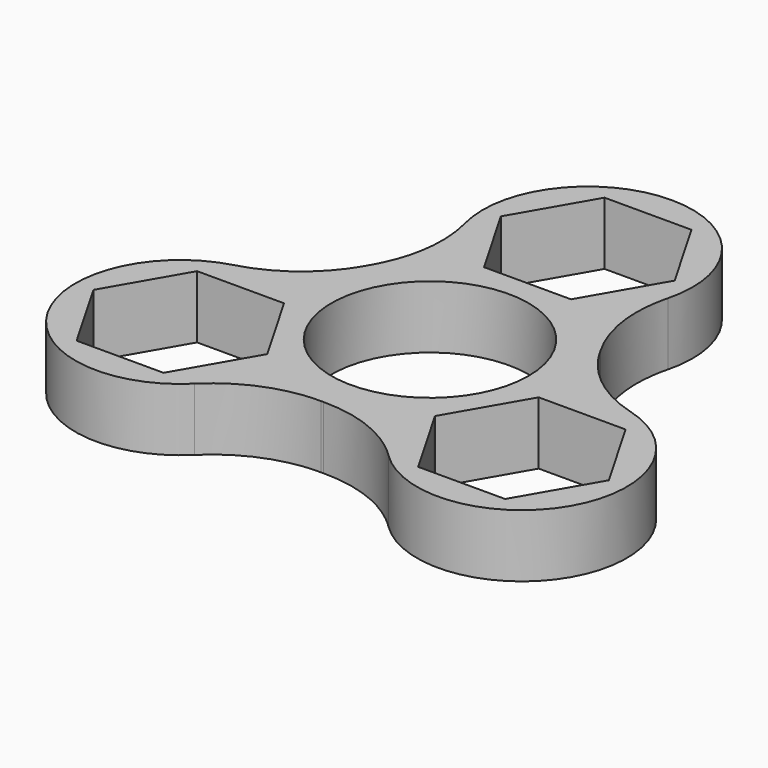
from build123d import *

# Parameters (mm, degrees)
F0_R     = 11
F1_DEPTH = 7
F2_R     = 15


with BuildPart() as f1:
    # F0 (on Top) → F1 (new body)
    with BuildSketch(Plane.XY):
        with BuildLine():
            ThreePointArc((-14.7729482501, -2.6), (-14.9420444362, -1.3173109227), (-14.9999794627, -0.0248217267))
            ThreePointArc((-14.9999794627, -0.0248217267), (-29.1846096908, -16.8497422612), (-7.5214859773, -12.9779524076))
            ThreePointArc((-7.5214859773, -12.9779524076), (-8.6118469419, -12.2815346048), (-9.6381401749, -11.4937484734))
            Line((-9.6381401749, -11.4937484734), (-14.2028166221, -19.4))
            Line((-14.2028166221, -19.4), (-23.9023011445, -19.4))
            Line((-23.9023011445, -19.4), (-28.7520434056, -11))
            Line((-28.7520434056, -11), (-23.9023011445, -2.6))
            Line((-23.9023011445, -2.6), (-14.7729482501, -2.6))
        make_face()
        with BuildLine():
            ThreePointArc((14.9999794627, -0.0248217267), (14.9999948657, -0.0124108676), (15, 0))
            ThreePointArc((15, 0), (12.9841711765, 7.5107455595), (7.4784934854, 13.0027741343))
            ThreePointArc((7.4784934854, 13.0027741343), (6.3301974943, 13.5988455276), (5.1348080752, 14.0937484734))
            Line((5.1348080752, 14.0937484734), (4.8497422612, 13.6))
            Line((4.8497422612, 13.6), (-4.8497422612, 13.6))
            Line((-4.8497422612, 13.6), (-5.1348080752, 14.0937484734))
            ThreePointArc((-5.1348080752, 14.0937484734), (-6.3301974943, 13.5988455276), (-7.4784934854, 13.0027741343))
            ThreePointArc((-7.4784934854, 13.0027741343), (-12.9903810568, 7.5), (-14.9999794627, -0.0248217267))
            ThreePointArc((-14.9999794627, -0.0248217267), (-14.9420444362, -1.3173109227), (-14.7729482501, -2.6))
            Line((-14.7729482501, -2.6), (-14.2028166221, -2.6))
            Line((-14.2028166221, -2.6), (-9.3530743609, -11))
            Line((-9.3530743609, -11), (-9.6381401749, -11.4937484734))
            ThreePointArc((-9.6381401749, -11.4937484734), (-8.6118469419, -12.2815346048), (-7.5214859773, -12.9779524076))
            ThreePointArc((-7.5214859773, -12.9779524076), (0, -15), (7.5214859773, -12.9779524076))
            ThreePointArc((7.5214859773, -12.9779524076), (8.6118469419, -12.2815346048), (9.6381401749, -11.4937484734))
            Line((9.6381401749, -11.4937484734), (9.3530743609, -11))
            Line((9.3530743609, -11), (14.2028166221, -2.6))
            Line((14.2028166221, -2.6), (14.7729482501, -2.6))
            ThreePointArc((14.7729482501, -2.6), (14.9420444362, -1.3173109227), (14.9999794627, -0.0248217267))
        make_face()
        Circle(F0_R, mode=Mode.SUBTRACT)
        with BuildLine():
            ThreePointArc((7.5214859773, -12.9779524076), (29.1846096908, -16.8497422612), (14.9999794627, -0.0248217267))
            ThreePointArc((14.9999794627, -0.0248217267), (14.9420444362, -1.3173109227), (14.7729482501, -2.6))
            Line((14.7729482501, -2.6), (23.9023011445, -2.6))
            Line((23.9023011445, -2.6), (28.7520434056, -11))
            Line((28.7520434056, -11), (23.9023011445, -19.4))
            Line((23.9023011445, -19.4), (14.2028166221, -19.4))
            Line((14.2028166221, -19.4), (9.6381401749, -11.4937484734))
            ThreePointArc((9.6381401749, -11.4937484734), (8.6118469419, -12.2815346048), (7.5214859773, -12.9779524076))
        make_face()
        with BuildLine():
            ThreePointArc((5.1348080752, 14.0937484734), (6.3301974943, 13.5988455276), (7.4784934854, 13.0027741343))
            ThreePointArc((7.4784934854, 13.0027741343), (0, 33.6994845224), (-7.4784934854, 13.0027741343))
            ThreePointArc((-7.4784934854, 13.0027741343), (-6.3301974943, 13.5988455276), (-5.1348080752, 14.0937484734))
            Line((-5.1348080752, 14.0937484734), (-9.6994845224, 22))
            Line((-9.6994845224, 22), (-4.8497422612, 30.4))
            Line((-4.8497422612, 30.4), (4.8497422612, 30.4))
            Line((4.8497422612, 30.4), (9.6994845224, 22))
            Line((9.6994845224, 22), (5.1348080752, 14.0937484734))
        make_face()
    extrude(amount=F1_DEPTH)

    # F2
    f2_edges = [f1.edges().sort_by_distance(p)[0] for p in [
        (7.521486, -12.977952, 3.5),
        (-14.999979, -0.024822, 3.5),
        (7.478493, 13.002774, 3.5),
        (-7.521486, -12.977952, 3.5),
        (14.999979, -0.024822, 3.5),
        (-7.478493, 13.002774, 3.5),
    ]]
    fillet(f2_edges, radius=F2_R)


solid = f1.part
